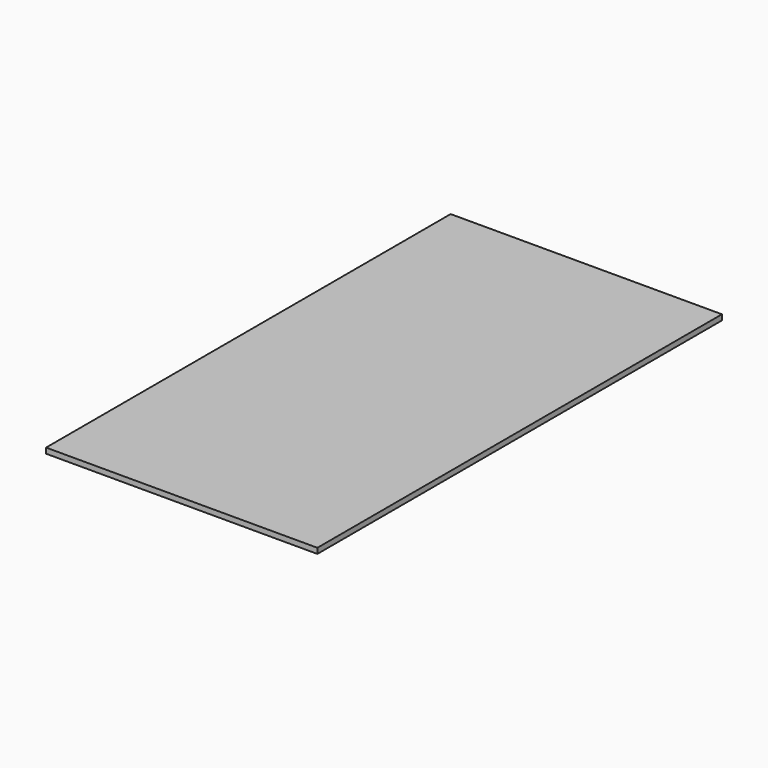
from build123d import *

# Parameters (mm, degrees)
F0_W     = 158.75
F0_H     = 295.91
F1_DEPTH = 3.175


# Not quite as in the source:
# - a length typed as a fraction of an inch, garbled in the dataset ("3 / 203.2 mm" for 3/8 in), is restored


with BuildPart() as f1:
    # F0 (on Top) → F1 (new body)
    with BuildSketch(Plane.XY):
        Rectangle(F0_W, F0_H)
    extrude(amount=F1_DEPTH)


solid = f1.part
